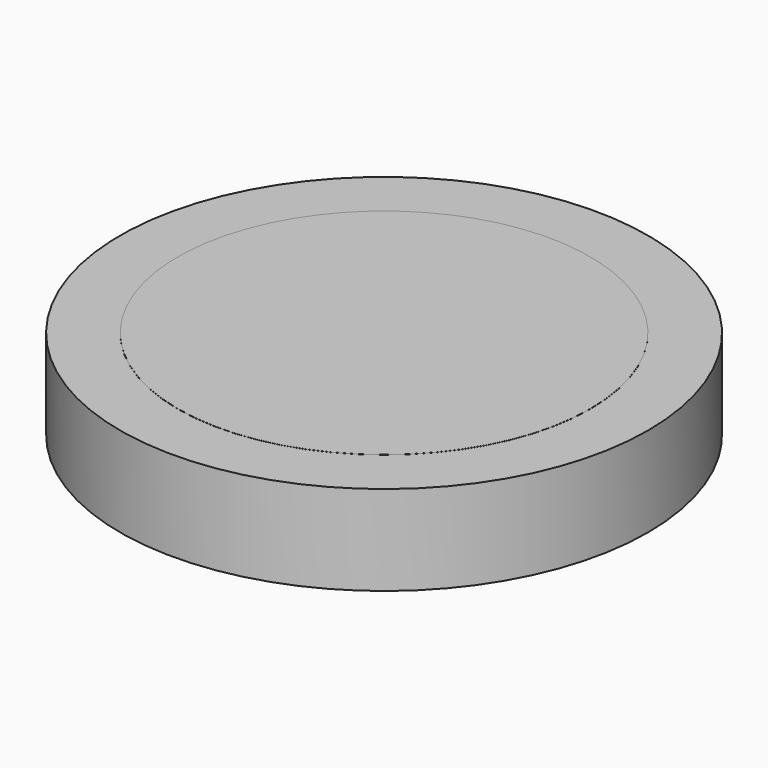
from build123d import *

# Parameters (mm, degrees)
F0_W = 13.434972614
F0_H = 20.8462406445


# Not quite as in the source:
# - ends of sketch curves that miss each other by under 0.0002 mm in the source are joined


with BuildPart() as f1:
    # F0 (on Front) → F1 (revolve)
    with BuildSketch(Plane.XZ):
        with BuildLine():
            ThreePointArc((31.0491894541, 4.37e-08), (37.0661020279, -6.0169125301), (43.0830146017, 4.37e-08))
            Line((43.0830146017, 4.37e-08), (31.0491894541, 4.37e-08))
        make_face()
        with Locations((54.5795354992, 10.4231199002)):
            Rectangle(F0_W, F0_H)
        with BuildLine():
            Line((31.0491894541, 4.37e-08), (43.0830146017, 4.37e-08))
            ThreePointArc((43.0830146017, 4.37e-08), (37.0661020279, 6.0169126175), (31.0491894541, 4.37e-08))
        make_face()
        with BuildLine():
            Line((47.8620491922, 20.8721738309), (0, 20.8721738309))
            Line((0, 20.8721738309), (0, 4.37e-08))
            Line((0, 4.37e-08), (4.3250534176, 4.37e-08))
            ThreePointArc((4.3250534176, 4.37e-08), (9.7163589671, 5.3913055932), (15.1076645166, 4.37e-08))
            Line((15.1076645166, 4.37e-08), (31.0491894541, 4.37e-08))
            ThreePointArc((31.0491894541, 4.37e-08), (37.0661020279, 6.0169126175), (43.0830146017, 4.37e-08))
            Line((43.0830146017, 4.37e-08), (47.8620491922, 4.37e-08))
            Line((47.8620491922, 4.37e-08), (47.8620491922, 20.8462402225))
            Line((47.8620491922, 20.8462402225), (47.8620491922, 20.8721738309))
        make_face()
        with BuildLine():
            ThreePointArc((15.1076645166, 4.37e-08), (9.7163589671, 5.3913055932), (4.3250534176, 4.37e-08))
            Line((4.3250534176, 4.37e-08), (15.1076645166, 4.37e-08))
        make_face()
        with BuildLine():
            Line((15.1076645166, 4.37e-08), (4.3250534176, 4.37e-08))
            ThreePointArc((4.3250534176, 4.37e-08), (9.7163589671, -5.3913055058), (15.1076645166, 4.37e-08))
        make_face()
    revolve(axis=Axis((0, 0, 10.4360869373), (0, 0, -1)))


solid = f1.part
